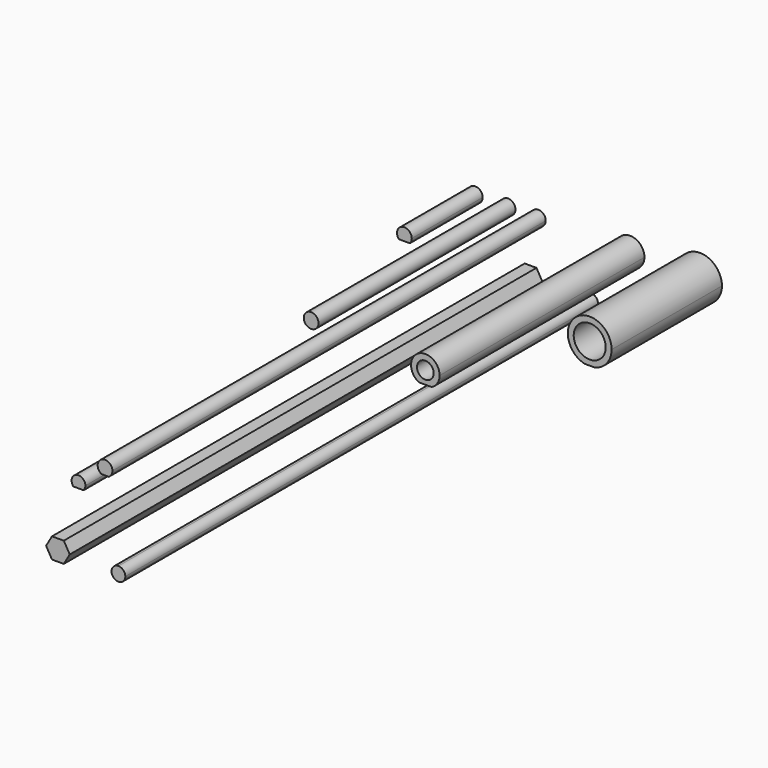
from build123d import *

# Parameters (mm, degrees)
F1_DEPTH = 18
F0_R     = 1.5
F2_DEPTH = 50
F3_DEPTH = 110
F4_DEPTH = 100
F0_R_2   = 1.7
F5_DEPTH = 52
F0_R_3   = 3.25
F6_DEPTH = 28
F7_DEPTH = 120
F8_DEPTH = 5
F9_DEPTH = 5


# Not quite as in the source:
# - a feature names something its author has since deleted; it is built from what else it names


with BuildPart() as f1:
    # F0 (on Front) → F1 (new body)
    with BuildSketch(Plane.XZ):
        with BuildLine():
            ThreePointArc((-8.5876567433, -1), (-8.3044321936, -0.5352331347), (-8.205690732, 0))
            ThreePointArc((-8.205690732, 0), (-10.2409238667, 1.4012585384), (-10.8237247208, -1))
            Line((-10.8237247208, -1), (-8.5876567433, -1))
        make_face()
    extrude(amount=F1_DEPTH)


with BuildPart() as f2:
    # F0 (on Front) → F2 (new body)
    with BuildSketch(Plane.XZ):
        with Locations((-3.0406215228, 0)):
            Circle(F0_R)
    extrude(amount=F2_DEPTH)


with BuildPart() as f3:
    # F0 (on Front) → F3 (new body)
    with BuildSketch(Plane.XZ):
        with BuildLine():
            ThreePointArc((4.6031738035, 0), (2.3531738035, 1.2990381057), (2.3531738035, -1.2990381057))
            Line((2.3531738035, -1.2990381057), (3.8531738035, -1.2990381057))
            ThreePointArc((3.8531738035, -1.2990381057), (4.4022119092, -0.75), (4.6031738035, 0))
        make_face()
    extrude(amount=F3_DEPTH)


with BuildPart() as f4:
    # F0 (on Front) → F4 (new body)
    with BuildSketch(Plane.XZ):
        with BuildLine():
            ThreePointArc((-9.2458325086, -12.0397212359), (-8.9814895955, -11.6059388283), (-8.8893308981, -11.1063879026))
            ThreePointArc((-8.8893308981, -11.1063879026), (-10.7888818238, -9.7985466), (-11.3328292876, -12.0397212359))
            Line((-11.3328292876, -12.0397212359), (-9.2458325086, -12.0397212359))
        make_face()
    extrude(amount=F4_DEPTH)


with BuildPart() as f5:
    # F0 (on Front) → F5 (new body)
    with BuildSketch(Plane.XZ):
        with BuildLine():
            ThreePointArc((23.0335708203, -2.6), (24.2122890699, -1.5305036021), (24.6490475625, 0))
            ThreePointArc((24.6490475625, 0), (20.2185439604, 2.4632415074), (20.4645243046, -2.6))
            Line((20.4645243046, -2.6), (23.0335708203, -2.6))
        make_face()
        with Locations((21.7490475625, 0)):
            Circle(F0_R_2, mode=Mode.SUBTRACT)
    extrude(amount=F5_DEPTH)


with BuildPart() as f6:
    # F0 (on Front) → F6 (new body)
    with BuildSketch(Plane.XZ):
        with BuildLine():
            ThreePointArc((36.9349649165, -4.3361849592), (39.4172414707, -2.7706046272), (40.3849649165, 0))
            ThreePointArc((40.3849649165, 0), (33.1643602893, 3.4822765542), (34.9349649165, -4.3361849592))
            Line((34.9349649165, -4.3361849592), (36.9349649165, -4.3361849592))
        make_face()
        with Locations((35.9349649165, 0)):
            Circle(F0_R_3, mode=Mode.SUBTRACT)
    extrude(amount=F6_DEPTH)


with BuildPart() as f7:
    # F0 (on Front) → F7 (new body)
    with BuildSketch(Plane.XZ):
        with BuildLine():
            ThreePointArc((13.8214863837, -12.754113929), (14.8114358773, -12.3440634226), (15.2214863837, -11.354113929))
            ThreePointArc((15.2214863837, -11.354113929), (14.8114358773, -10.3641644353), (13.8214863837, -9.954113929))
            ThreePointArc((13.8214863837, -9.954113929), (12.83153689, -10.3641644353), (12.4214863837, -11.354113929))
            ThreePointArc((12.4214863837, -11.354113929), (12.83153689, -12.3440634226), (13.8214863837, -12.754113929))
        make_face()
    extrude(amount=F7_DEPTH)

    # F0 (on Front) → F9 (join)
    with BuildSketch(Plane.XZ):
        with BuildLine():
            Line((12.4214863837, -12.754113929), (13.8214863837, -12.754113929))
            ThreePointArc((13.8214863837, -12.754113929), (12.83153689, -12.3440634226), (12.4214863837, -11.354113929))
            Line((12.4214863837, -11.354113929), (12.4214863837, -12.754113929))
        make_face()
        with BuildLine():
            Line((15.2214863837, -12.754113929), (15.2214863837, -11.354113929))
            ThreePointArc((15.2214863837, -11.354113929), (14.8114358773, -12.3440634226), (13.8214863837, -12.754113929))
            Line((13.8214863837, -12.754113929), (15.2214863837, -12.754113929))
        make_face()
    extrude(amount=F9_DEPTH)


with BuildPart() as f7b:
    # F0 (on Front) → F7, piece 2 (new body)
    with BuildSketch(Plane.XZ):
        Polygon((2.7269763106, -13.1848488717), (3.9269763106, -11.1063879026), (2.7269763106, -9.0279269335), (0.3269763106, -9.0279269335), (-0.8730236894, -11.1063879026), (0.3269763106, -13.1848488717), align=None)
    extrude(amount=F7_DEPTH)

    # F0 (on Front) → F8 (join)
    with BuildSketch(Plane.XZ):
        with BuildLine():
            Line((-0.8730236894, -13.1848488717), (0.3269763106, -13.1848488717))
            ThreePointArc((0.3269763106, -13.1848488717), (-0.5514846585, -12.3063879026), (-0.8730236894, -11.1063879026))
            Line((-0.8730236894, -11.1063879026), (-0.8730236894, -13.1848488717))
        make_face()
        with BuildLine():
            Line((3.9269763106, -13.1848488717), (3.9269763106, -11.1063879026))
            ThreePointArc((3.9269763106, -11.1063879026), (3.6054372797, -12.3063879026), (2.7269763106, -13.1848488717))
            Line((2.7269763106, -13.1848488717), (3.9269763106, -13.1848488717))
        make_face()
        with BuildLine():
            ThreePointArc((2.7269763106, -13.1848488717), (3.6054372797, -12.3063879026), (3.9269763106, -11.1063879026))
            Line((3.9269763106, -11.1063879026), (2.7269763106, -13.1848488717))
        make_face()
        with BuildLine():
            ThreePointArc((-0.8730236894, -11.1063879026), (-0.5514846585, -12.3063879026), (0.3269763106, -13.1848488717))
            Line((0.3269763106, -13.1848488717), (-0.8730236894, -11.1063879026))
        make_face()
    extrude(amount=F8_DEPTH)


solid = Compound([f1.part, f2.part, f3.part, f4.part, f5.part, f6.part, f7.part, f7b.part])
